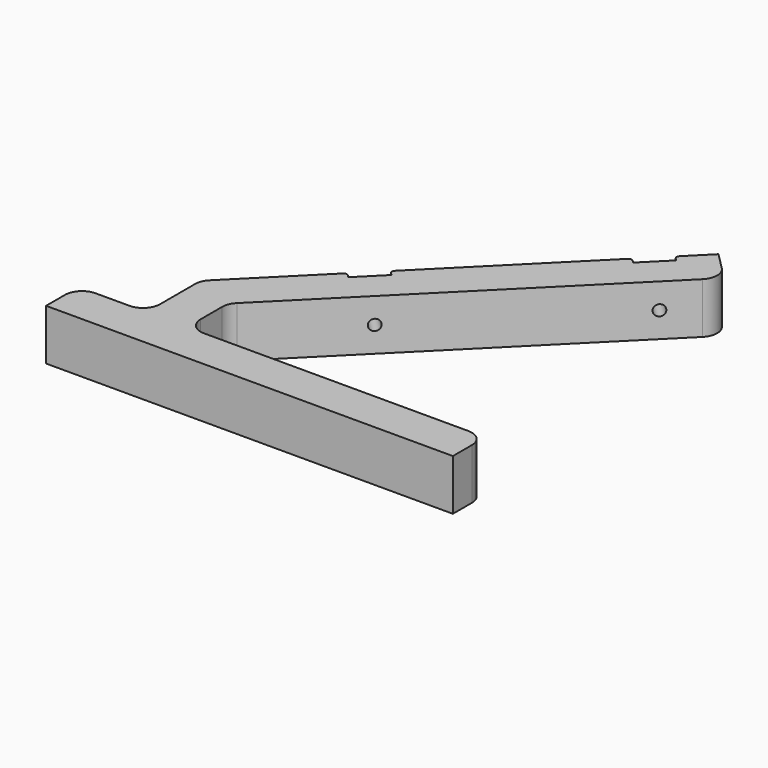
from build123d import *

# Parameters (mm, degrees)
F1_DEPTH = 15
F2_R     = 5
F3_W     = 10
F3_H     = 15
F4_DEPTH = 2
F5_D     = 3.2
F5_DEPTH = 25
F5_TIP   = 0.9613769904
F6_R     = 1


with BuildPart() as f1:
    # F0 (on Top) → F1 (new body)
    with BuildSketch(Plane.XY):
        Polygon((-40, 6), (-28, 6), (-28, 21.0294372515), (53.3380951166, 102.3675323681), (44.8528137424, 110.8528137424), (-40, 26), align=None)
        Polygon((-60, -6), (60, -6), (60, 6), (-28, 6), (-40, 6), (-60, 6), align=None)
    extrude(amount=F1_DEPTH)

    # F2
    f2_edges = [f1.edges().sort_by_distance(p)[0] for p in [
        (-40, 6, 7.5),
        (-28, 6, 7.5),
        (-60, 6, 7.5),
        (60, 6, 7.5),
        (53.338095, 102.367532, 7.5),
        (-40, 26, 7.5),
        (-28, 21.029437, 7.5),
    ]]
    fillet(f2_edges, radius=F2_R)

    # F3 (on face) → F4 (cut)
    with BuildSketch(Plane(origin=(-33, 33, 0), x_dir=(-0.7071067812, -0.7071067812, 0), z_dir=(-0.7071067812, 0.7071067812, 0))):
        with Locations((-95.1005050634, 7.5)):
            Rectangle(F3_W, F3_H)
        with Locations((-29.1005050634, 7.5)):
            Rectangle(F3_W, F3_H)
    extrude(amount=-F4_DEPTH, mode=Mode.SUBTRACT)

    # F5
    with Locations(Plane(origin=(-33, 33, 0), x_dir=(-0.7071067812, -0.7071067812, 0), z_dir=(-0.7071067812, 0.7071067812, 0))):
        with Locations((-95.1005050634, 7.5), (-29.1005050634, 7.5)):
            Hole(F5_D / 2, depth=F5_DEPTH)
            with Locations((0, 0, -(F5_DEPTH + F5_TIP / 2))):  # 118° drill point
                Cone(0, F5_D / 2, F5_TIP, mode=Mode.SUBTRACT)

    # F6
    f6_edges = [f1.edges().sort_by_distance(p)[0] for p in [
        (37.781746, 103.781746, 7.5),
        (30.710678, 96.710678, 7.5),
        (-8.887302, 57.112698, 7.5),
        (-15.958369, 50.041631, 7.5),
    ]]
    fillet(f6_edges, radius=F6_R)


solid = f1.part
